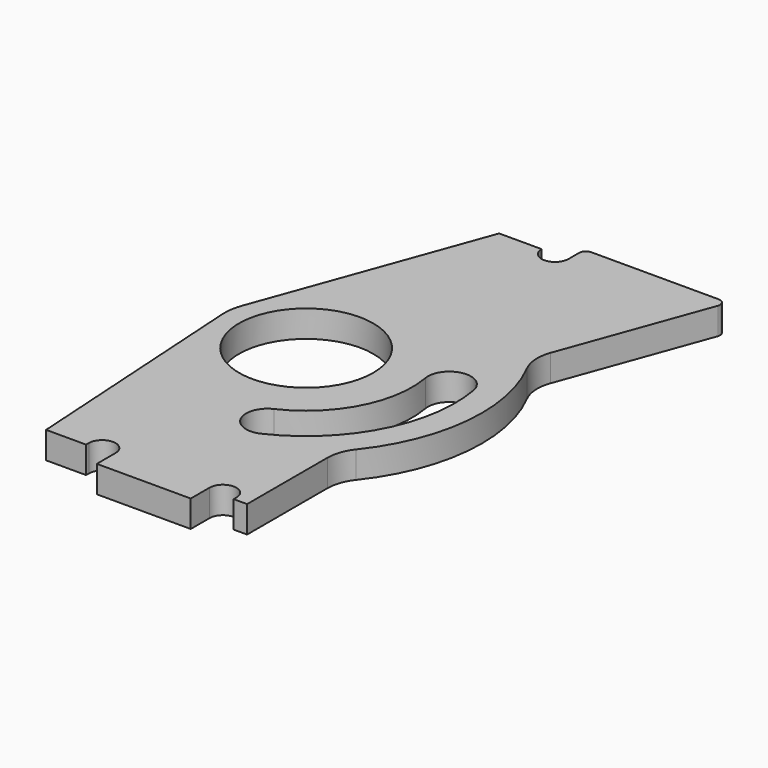
from build123d import *

# Parameters (mm, degrees)
F0_R     = 5
F1_DEPTH = 2


# Not quite as in the source:
# - ends of sketch curves that miss each other by under 0.0002 mm in the source are joined


with BuildPart() as f1:
    # F0 (on Top) → F1 (new body)
    with BuildSketch(Plane.XY):
        with BuildLine():
            ThreePointArc((7.1735815028, 5.6201217427), (6.8442176511, 6.8062722819), (7.0189573047, 8.0248368891))
            Line((7.0189573047, 8.0248368891), (10.91495, 18.72899))
            ThreePointArc((10.91495, 18.72899), (10.8546800333, 19.1867882023), (10.445104, 19.4))
            Line((10.445104, 19.4), (0.946042, 19.4))
            ThreePointArc((0.946042, 19.4), (0.5924886094, 19.2535533906), (0.446042, 18.9))
            Line((0.446042, 18.9), (0.446042, 17.9))
            ThreePointArc((0.446042, 17.9), (-0.553958, 16.9), (-1.553958, 17.9))
            Line((-1.553958, 17.9), (-4.717745, 17.9))
            Line((-4.717745, 17.9), (-10.704846, 1.450575))
            ThreePointArc((-10.704846, 1.450575), (-10.9040414443, 0.6585195076), (-10.9375317857, -0.1575129868))
            Line((-10.9375317857, -0.1575129868), (-9.842048, -17.9))
            Line((-9.842048, -17.9), (-6.861651, -17.9))
            Line((-6.861651, -17.9), (-6.861651, -17.65))
            ThreePointArc((-6.861651, -17.65), (-5.861651, -16.65), (-4.861651, -17.65))
            Line((-4.861651, -17.65), (-4.861651, -19.4))
            Line((-4.861651, -19.4), (2.138349, -19.4))
            Line((2.138349, -19.4), (2.138349, -17.65))
            ThreePointArc((2.138349, -17.65), (3.138349, -16.65), (4.138349, -17.65))
            Line((4.138349, -17.65), (4.138349, -17.9))
            Line((4.138349, -17.9), (5.138349, -17.9))
            Line((5.138349, -17.9), (5.138349, -10.423043))
            ThreePointArc((5.138349, -10.423043), (5.3061038311, -9.4339083765), (5.7906072022, -8.5553951609))
            ThreePointArc((5.7906072022, -8.5553951609), (8.5768989173, -1.6720073498), (7.1735815028, 5.6201217427))
        make_face()
        with Locations((-4.461199, -0.4)):
            Circle(F0_R, mode=Mode.SUBTRACT)
        with BuildLine():
            ThreePointArc((0.2298636534, -10.4600162566), (-1.8964183588, -9.6861134342), (-1.122515215, -7.559831539))
            ThreePointArc((-1.122515215, -7.559831539), (2.5461863518, -4.0478144871), (3.3187823445, 0.9718200607))
            ThreePointArc((3.3187823445, 0.9718200607), (4.6166380137, 2.8253494221), (6.470167407, 1.5274940718))
            ThreePointArc((6.470167407, 1.5274940718), (5.3846210817, -5.5254099269), (0.2298636534, -10.4600162566))
        make_face(mode=Mode.SUBTRACT)
    extrude(amount=F1_DEPTH)


solid = f1.part
